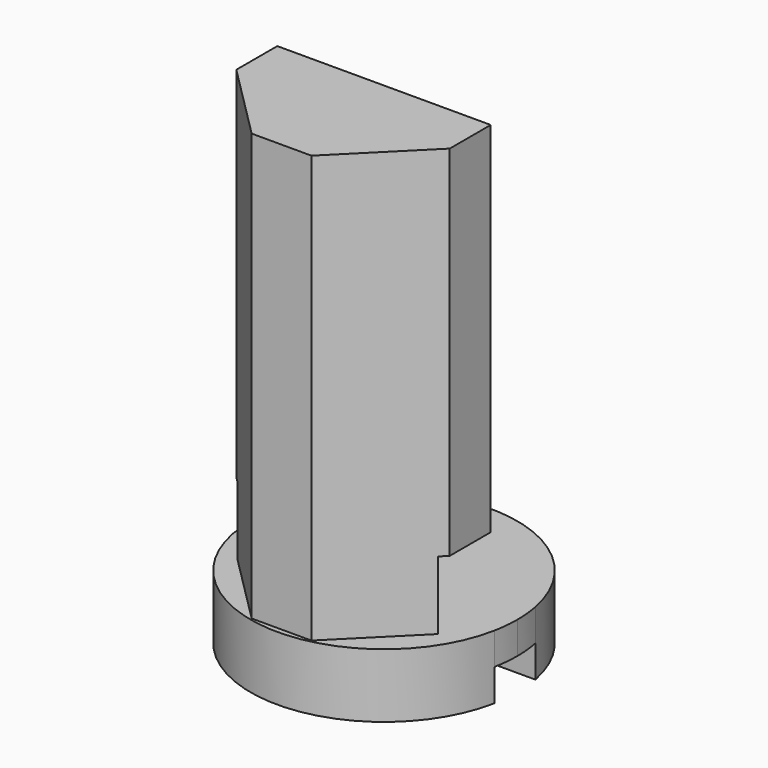
from build123d import *

# Parameters (mm, degrees)
F1_DEPTH      = 1.5
F2_DEPTH      = 0.75
F4_DEPTH      = 10
F5_T1_DEPTH   = 14.6290293783
F6_W          = 1.35
F6_H          = 1.6
F7_DEPTH      = 3.126
F7_DEPTH_BACK = 25
F9_DEPTH      = 0.75


# Not quite as in the source:
# - a fillet or chamfer that OpenCascade refuses, or shapes differently, is made with other operations: its cross-section is extruded or revolved along the edge and cut away or added


with BuildPart() as f1:
    # F0 (on Top) → F1 (new body)
    with BuildSketch(Plane.XY):
        with BuildLine():
            Line((-3.0668591425, 0.6), (3.0668591425, 0.6))
            ThreePointArc((3.0668591425, 0.6), (0, 3.125), (-3.0668591425, 0.6))
        make_face()
        with BuildLine():
            ThreePointArc((3.0668591425, -0.6), (3.1104308239, -0.3014051921), (3.125, 0))
            ThreePointArc((3.125, 0), (3.1104308239, 0.3014051921), (3.0668591425, 0.6))
            Line((3.0668591425, 0.6), (-3.0668591425, 0.6))
            ThreePointArc((-3.0668591425, 0.6), (-3.125, 0), (-3.0668591425, -0.6))
            Line((-3.0668591425, -0.6), (3.0668591425, -0.6))
        make_face()
        with BuildLine():
            ThreePointArc((-3.0668591425, -0.6), (0, -3.125), (3.0668591425, -0.6))
            Line((3.0668591425, -0.6), (-3.0668591425, -0.6))
        make_face()
    extrude(amount=F1_DEPTH)

    # F0 (on Top) → F2 (cut)
    with BuildSketch(Plane.XY):
        with BuildLine():
            ThreePointArc((3.0668591425, -0.6), (3.1104308239, -0.3014051921), (3.125, 0))
            ThreePointArc((3.125, 0), (3.1104308239, 0.3014051921), (3.0668591425, 0.6))
            Line((3.0668591425, 0.6), (-3.0668591425, 0.6))
            ThreePointArc((-3.0668591425, 0.6), (-3.125, 0), (-3.0668591425, -0.6))
            Line((-3.0668591425, -0.6), (3.0668591425, -0.6))
        make_face()
    extrude(amount=F2_DEPTH, mode=Mode.SUBTRACT)

    # F3 (on face) → F4 (join)
    with BuildSketch(Plane.XY.offset(1.5)):
        with BuildLine():
            ThreePointArc((-0.875, -3), (-1.7787811838, -2.5693505989), (-2.5, -1.875))
            Line((-2.5, -1.875), (-2.5, -3))
            Line((-2.5, -3), (-0.875, -3))
        make_face()
        with BuildLine():
            Line((2.5, 0), (-2.5, 0))
            Line((-2.5, 0), (-2.5, -1.875))
            ThreePointArc((-2.5, -1.875), (-1.7787811838, -2.5693505989), (-0.875, -3))
            Line((-0.875, -3), (0.875, -3))
            ThreePointArc((0.875, -3), (1.7787811838, -2.5693505989), (2.5, -1.875))
            Line((2.5, -1.875), (2.5, 0))
        make_face()
        with BuildLine():
            Line((2.5, -3), (2.5, -1.875))
            ThreePointArc((2.5, -1.875), (1.7787811838, -2.5693505989), (0.875, -3))
            Line((0.875, -3), (2.5, -3))
        make_face()
    extrude(amount=F4_DEPTH)

    # F5: chamfer of 1.8 on 2 edges, made by hand

    # F5_s2 → F5_t1 (cut)
    with BuildSketch(Plane.XY.offset(1.5)):
        Polygon((-2.5, -1.2), (-0.7, -3), (-2.5, -3), align=None)
        Polygon((2.5, -1.2), (0.7, -3), (2.5, -3), align=None)
    extrude(amount=F5_T1_DEPTH, mode=Mode.SUBTRACT)

    # F6 (on Right) → F7 (cut, two sides)
    with BuildSketch(Plane.YZ) as f7_sk:
        with Locations((-0.675, 2.3)):
            Rectangle(F6_W, F6_H)
    extrude(amount=-F7_DEPTH, mode=Mode.SUBTRACT)
    extrude(f7_sk.sketch, amount=F7_DEPTH_BACK, mode=Mode.SUBTRACT)

    # F8 (on Right) → F9 (join, symmetric)
    with BuildSketch(Plane.YZ):
        Polygon((0, 5.1), (0, 3.1), (1.2, 3.1), align=None)
    extrude(amount=F9_DEPTH, both=True)


solid = f1.part
